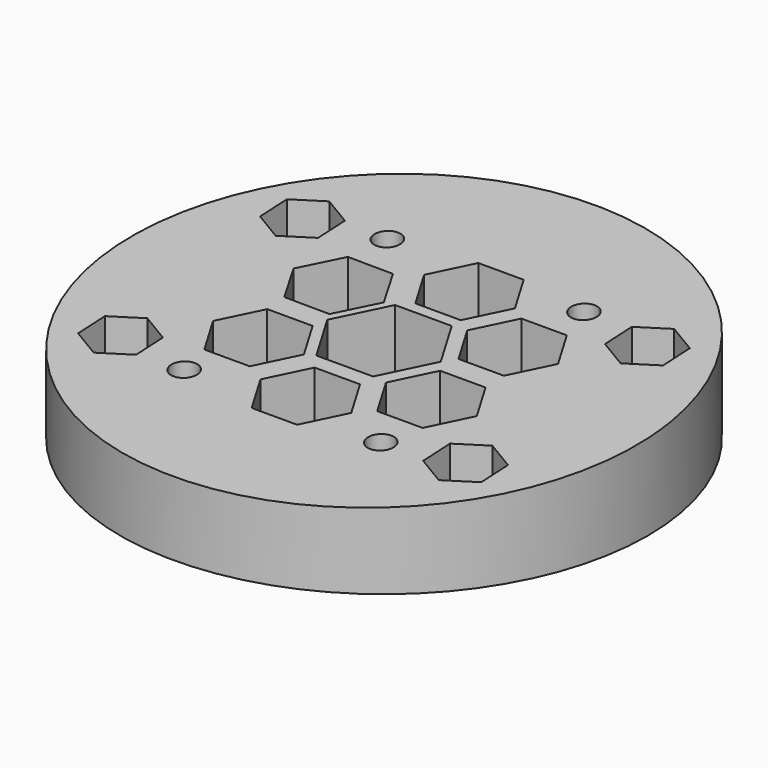
from build123d import *

# Parameters (mm, degrees)
F0_R      = 40.2650795079
F0_R_2    = 2
F2_DEPTH  = 20
F4_DEPTH  = 69.8
F6_DEPTH  = 25.001
F7_DEPTH  = 5
F8_R      = 2.5
F9_DEPTH  = 14.9319422489
F11_DEPTH = 13


# Not quite as in the source:
# - a feature names something its author has since deleted; it is built from what else it names


with BuildPart() as f2:
    # F0 (on Top) → F2 (new body)
    with BuildSketch(Plane.XY):
        with Locations((-11.4915669638, 7.0636273592)):
            Circle(F0_R)
        with Locations((-26.4915669638, -12.3077432686)):
            Circle(F0_R_2, mode=Mode.SUBTRACT)
        with Locations((3.5084330362, -12.3077432686)):
            Circle(F0_R_2, mode=Mode.SUBTRACT)
        with Locations((-26.4915669638, 26.434997987)):
            Circle(F0_R_2, mode=Mode.SUBTRACT)
        with Locations((3.5084330362, 26.434997987)):
            Circle(F0_R_2, mode=Mode.SUBTRACT)
    extrude(amount=F2_DEPTH)

    # F3 (on Right) → F4 (cut, symmetric)
    with BuildSketch(Plane.YZ):
        Polygon((-43.8041239977, 30.4956686149), (-39.6489202976, 15.9488338977), (68.1266114116, 20.8831354976), (67.6865195207, 30.4956686149), align=None)
    extrude(amount=F4_DEPTH, both=True, mode=Mode.SUBTRACT)

    # F5 (on offset) → F6 (cut, through all)
    with BuildSketch(Plane.XY.offset(25)):
        Polygon((-4.9963764354, 14.8136273592), (-1.5322748203, 8.8136273592), (5.39592841, 8.8136273592), (8.8600300251, 14.8136273592), (5.39592841, 20.8136273592), (-1.5322748203, 20.8136273592), align=None)
        Polygon((-1.5322748203, 5.3136273592), (-4.9963764354, -0.6863726408), (-1.5322748203, -6.6863726408), (5.39592841, -6.6863726408), (8.8600300251, -0.6863726408), (5.39592841, 5.3136273592), align=None)
        Polygon((-14.170220135, -2.8258145228), (-17.6343217501, -8.8258145228), (-14.170220135, -14.8258145228), (-7.2420169047, -14.8258145228), (-3.7779152896, -8.8258145228), (-7.2420169047, -2.8258145228), align=None)
        Polygon((-27.5721969216, 4.890474733), (-31.0362985367, -1.109525267), (-27.5721969216, -7.109525267), (-20.6439936913, -7.109525267), (-17.1798920761, -1.109525267), (-20.6439936913, 4.890474733), align=None)
        Polygon((-7.1614399449, 14.5636273592), (-15.8216939827, 14.5636273592), (-20.1518210017, 7.0636273592), (-15.8216939827, -0.4363726408), (-7.1614399449, -0.4363726408), (-2.831312926, 7.0636273592), align=None)
        Polygon((-27.6414862443, 20.3495556396), (-31.1520113303, 14.3765987822), (-27.7345414991, 8.3499164484), (-20.8065465819, 8.296190972), (-17.2960214958, 14.2691478294), (-20.7134913271, 20.2958301632), align=None)
        Polygon((-14.0889966993, 28.28301467), (-17.5530983144, 22.28301467), (-14.0889966993, 16.28301467), (-7.160793469, 16.28301467), (-3.6966918539, 22.28301467), (-7.160793469, 28.28301467), align=None)
    extrude(amount=-F6_DEPTH, mode=Mode.SUBTRACT)

    # F7 (cut): a face of the model
    f7_faces = [f2.faces().sort_by_distance(p)[0] for p in [
        (-50.6177780411, 7.0636273592, 0),
    ]]
    extrude(f7_faces, amount=-F7_DEPTH, mode=Mode.SUBTRACT)

    # F8 (on face) → F9 (cut, through all)
    with BuildSketch(Plane(origin=(0, 0, 5), x_dir=(1, 0, 0), z_dir=(0, 0, -1))):
        with Locations((14.8332985118, 10.2885384113)):
            Circle(F8_R)
        with Locations((14.8332985118, -24.3908837438)):
            Circle(F8_R)
        with Locations((-37.8164324394, -24.4157931297)):
            Circle(F8_R)
        with Locations((-37.8164324394, 10.2885384113)):
            Circle(F8_R)
    extrude(amount=-F9_DEPTH, mode=Mode.SUBTRACT)

    # F10 (on offset) → F11 (cut)
    with BuildSketch(Plane.XY.offset(25)):
        Polygon((19.2582985118, -12.8433133524), (19.2582985118, -7.7337634701), (14.8332985118, -5.1789885289), (10.4082985118, -7.7337634701), (10.4082985118, -12.8433133524), (14.8332985118, -15.3980882936), align=None)
        Polygon((19.2582985118, 21.8361088026), (19.2582985118, 26.9456586849), (14.8332985118, 29.5004336261), (10.4082985118, 26.9456586849), (10.4082985118, 21.8361088026), (14.8332985118, 19.2813338614), align=None)
        Polygon((-33.3914324394, 21.8610181886), (-33.3914324394, 26.9705680709), (-37.8164324394, 29.5253430121), (-42.2414324394, 26.9705680709), (-42.2414324394, 21.8610181886), (-37.8164324394, 19.3062432474), align=None)
        Polygon((-33.3914324394, -12.8433133524), (-33.3914324394, -7.7337634701), (-37.8164324394, -5.1789885289), (-42.2414324394, -7.7337634701), (-42.2414324394, -12.8433133524), (-37.8164324394, -15.3980882936), align=None)
    extrude(amount=-F11_DEPTH, mode=Mode.SUBTRACT)


solid = f2.part
